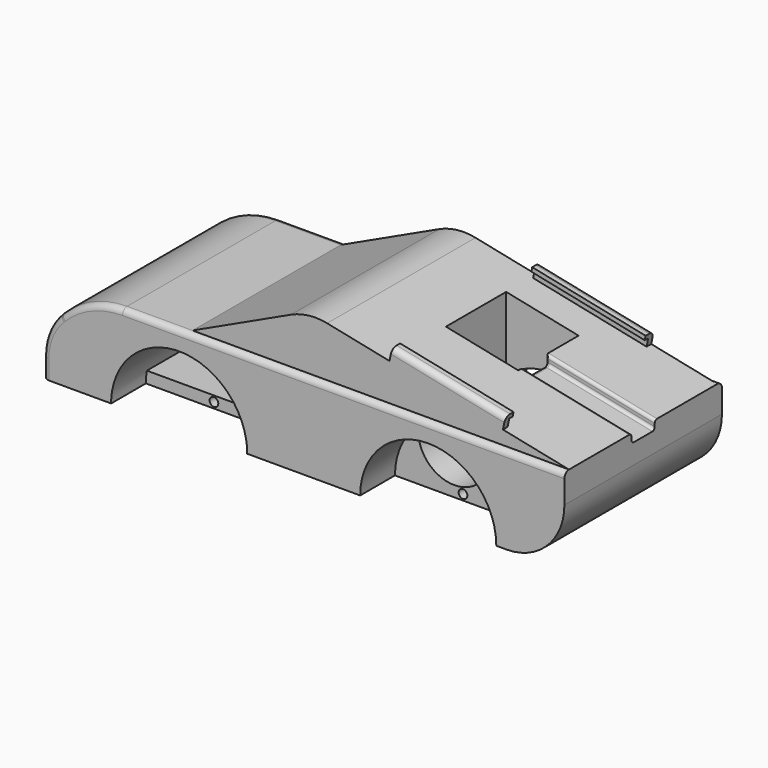
from build123d import *

# Parameters (mm, degrees)
F1_DEPTH       = 34
F2_DEPTH       = 32
F0_R           = 1.5
F3_DEPTH       = 19
F4_R           = 12.5
F5_DEPTH       = 38
F7_W           = 25
F7_H           = 26
F8_DEPTH       = 32.4283063262
F9_R           = 20
F10_R          = 30
F11_R          = 1.99999
F12_R          = 20
F15_DEPTH      = 15
F15_DEPTH_BACK = 25
F16_R          = 2
F17_W          = 10
F17_H          = 6
F18_DEPTH      = 40
F19_R          = 1


# Not quite as in the source:
# - a fillet or chamfer is up to 0.001 mm smaller than in the source, because OpenCascade refuses the exact size


with BuildPart() as f1:
    # F0 (on Front) → F1 (new body, symmetric)
    with BuildSketch(Plane.XZ):
        with BuildLine():
            Line((90, -15), (90, 15))
            Line((90, 15), (-40, 15))
            Line((-40, 15), (-75, 15))
            Line((-75, 15), (-90, 0))
            Line((-90, 0), (-90, -15))
            Line((-90, -15), (-66.5, -15))
            ThreePointArc((-66.5, -15), (-66.4141111332, -12.9926634954), (-66.1570723538, -11))
            ThreePointArc((-66.1570723538, -11), (-43, 8.5), (-19.8429276462, -11))
            ThreePointArc((-19.8429276462, -11), (-19.5858888668, -12.9926634954), (-19.5, -15))
            Line((-19.5, -15), (19.5, -15))
            ThreePointArc((19.5, -15), (21.6186797268, -5.2486337688), (27.5926930532, 2.7444327226))
            ThreePointArc((27.5926930532, 2.7444327226), (37.7272727273, 13.516632815), (51.0436705831, 7.0805200018))
            ThreePointArc((51.0436705831, 7.0805200018), (62.2519642985, -1.5236551451), (66.5, -15))
            Line((66.5, -15), (90, -15))
        make_face()
        with BuildLine():
            ThreePointArc((27.5926930532, 2.7444327226), (38.7272727273, 8.1083059018), (51.0436705831, 7.0805200018))
            ThreePointArc((51.0436705831, 7.0805200018), (37.7272727273, 13.516632815), (27.5926930532, 2.7444327226))
        make_face()
    extrude(amount=F1_DEPTH, both=True)

    # F0 (on Front) → F2 (join, symmetric)
    with BuildSketch(Plane.XZ):
        Polygon((-40, 15), (90, 15), (0, 33.6523063262), align=None)
    extrude(amount=F2_DEPTH, both=True)

    # F0 (on Front) → F3 (join, symmetric)
    with BuildSketch(Plane.XZ):
        with BuildLine():
            Line((-66.5, -15), (-19.5, -15))
            ThreePointArc((-19.5, -15), (-19.5858888668, -12.9926634954), (-19.8429276462, -11))
            Line((-19.8429276462, -11), (-66.1570723538, -11))
            ThreePointArc((-66.1570723538, -11), (-66.4141111332, -12.9926634954), (-66.5, -15))
        make_face()
        with Locations((-43, -13)):
            Circle(F0_R, mode=Mode.SUBTRACT)
        with BuildLine():
            Line((19.5, -15), (66.5, -15))
            ThreePointArc((66.5, -15), (62.2519642985, -1.5236551451), (51.0436705831, 7.0805200018))
            ThreePointArc((51.0436705831, 7.0805200018), (52.1304551087, 4.2419425981), (52.5, 1.2249807396))
            ThreePointArc((52.5, 1.2249807396), (39.2388616534, -11.2518244772), (27.5926930532, 2.7444327226))
            ThreePointArc((27.5926930532, 2.7444327226), (21.6186797268, -5.2486337688), (19.5, -15))
        make_face()
        with Locations((43, -13)):
            Circle(F0_R, mode=Mode.SUBTRACT)
        with BuildLine():
            ThreePointArc((52.5, 1.2249807396), (52.1304551087, 4.2419425981), (51.0436705831, 7.0805200018))
            ThreePointArc((51.0436705831, 7.0805200018), (38.7272727273, 8.1083059018), (27.5926930532, 2.7444327226))
            ThreePointArc((27.5926930532, 2.7444327226), (39.2388616534, -11.2518244772), (52.5, 1.2249807396))
        make_face()
    extrude(amount=F3_DEPTH, both=True)

    # F4 (on face) → F5 (cut)
    with BuildSketch(Plane.XZ.offset(19)):
        with Locations((40, 1.2249807396)):
            Circle(F4_R)
    extrude(amount=-F5_DEPTH, mode=Mode.SUBTRACT)

    # F7 (on offset) → F8 (cut, through all)
    with BuildSketch(Plane.XY.offset(1.225)):
        with Locations((40, 6)):
            Rectangle(F7_W, F7_H)
    extrude(amount=F8_DEPTH, mode=Mode.SUBTRACT)

    # F9
    f9_edges = [f1.edges().sort_by_distance(p)[0] for p in [
        (0, 0, 33.652306),
        (-90, 0, 0),
    ]]
    fillet(f9_edges, radius=F9_R)

    # F10
    f10_edges = [f1.edges().sort_by_distance(p)[0] for p in [
        (-75, 0, 15),
    ]]
    fillet(f10_edges, radius=F10_R)

    # F11 (radius 2 in the source; OpenCascade refuses exactly that, so slightly less here)
    f11_edges = [f1.edges().sort_by_distance(p)[0] for p in [
        (13.713203, -34, 15),
        (13.713203, 34, 15),
    ]]
    fillet(f11_edges, radius=F11_R)

    # F12
    f12_edges = [f1.edges().sort_by_distance(p)[0] for p in [
        (90, 0, -15),
    ]]
    fillet(f12_edges, radius=F12_R)

    # F14 (on face) → F15 (join, two sides)
    with BuildSketch(Plane(origin=(45.8128559398, 0, -9.4946158074), x_dir=(0, 1, 0), z_dir=(0.9791921158, 0, -0.2029354588))) as f15_sk:
        Polygon((-32, 37.2520730314), (-32, 32.9520730314), (-30, 32.9520730314), (-30, 35.7520730314), (-28.5, 35.7520730314), (-28.5, 37.2520730314), align=None)
        Polygon((28.5, 35.7520730314), (30, 35.7520730314), (30, 32.9520730314), (32, 32.9520730314), (32, 37.2520730314), (28.5, 37.2520730314), align=None)
    extrude(amount=F15_DEPTH)
    extrude(f15_sk.sketch, amount=-F15_DEPTH_BACK)

    # F16
    f16_edges = [f1.edges().sort_by_distance(p)[0] for p in [
        (48.476662, -32, 27.996998),
        (48.476662, 32, 27.996998),
    ]]
    fillet(f16_edges, radius=F16_R)

    # F17 (on face) → F18 (cut)
    with BuildSketch(Plane(origin=(45.8128559398, 0, -9.4946158074), x_dir=(0, 1, 0), z_dir=(0.9791921158, 0, -0.2029354588))):
        with Locations((0, 32.9520730314)):
            Rectangle(F17_W, F17_H)
    extrude(amount=F18_DEPTH, mode=Mode.SUBTRACT)

    # F19
    f19_edges = [f1.edges().sort_by_distance(p)[0] for p in [
        (52.5, 0, 19.708044),
        (52.5, -5, 21.239919),
        (52.5, 5, 21.239919),
        (71.25, -5, 15.822147),
        (71.25, 5, 15.822147),
        (71.25, -5, 18.885897),
        (71.25, 5, 18.885897),
    ]]
    fillet(f19_edges, radius=F19_R)


solid = f1.part
